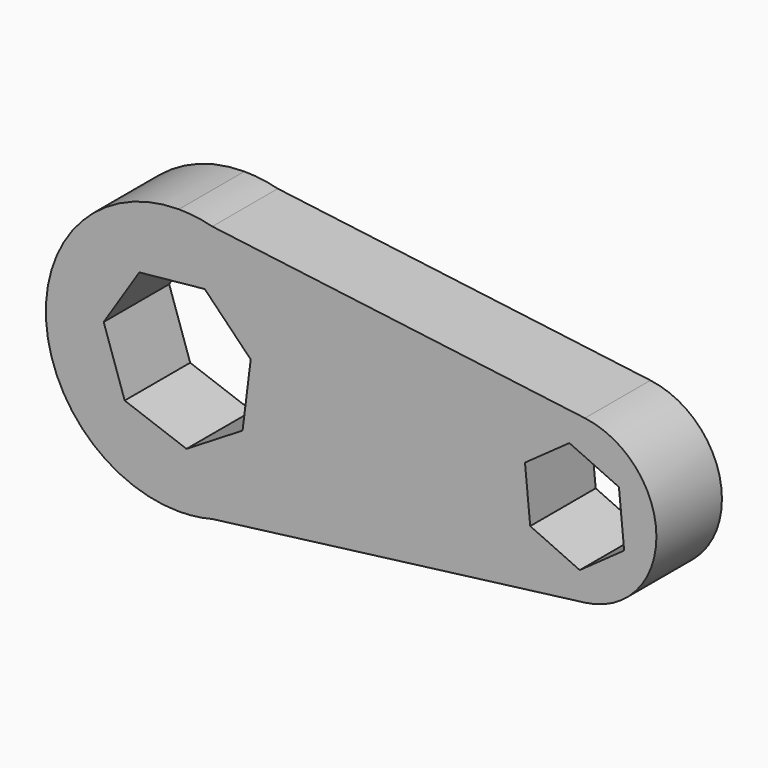
from build123d import *

# Parameters (mm, degrees)
F1_DEPTH = 50.8


# Not quite as in the source:
# - a feature names something its author has since deleted; it is built from what else it names


with BuildPart() as f1:
    # F0 (on Front) → F1 (new body)
    with BuildSketch(Plane.XZ):
        with BuildLine():
            Line((20.7350080501, 79.903453875), (0, 82.55))
            ThreePointArc((0, 82.55), (-82.55, 0), (0, -82.55))
            Line((0, -82.55), (20.7350080501, -79.903453875))
            ThreePointArc((20.7350080501, -79.903453875), (65.2923326836, -50.511521386), (82.55, 0))
            ThreePointArc((82.55, 0), (65.2923326836, 50.511521386), (20.7350080501, 79.903453875))
        make_face()
        Polygon((44.563520115, 15.0143387373), (39.5235830399, -25.4798759112), (4.7215818015, -46.7872243038), (-33.6358668361, -32.8628385102), (-46.6648216995, 5.8079349613), (-24.5542140343, 40.1052149467), (16.0462176134, 44.2024500799), align=None, mode=Mode.SUBTRACT)
        with BuildLine():
            ThreePointArc((20.7350080501, 79.903453875), (10.4516119, 81.8856905002), (0, 82.55))
            Line((0, 82.55), (20.7350080501, 79.903453875))
        make_face()
        with BuildLine():
            Line((20.7350080501, -79.903453875), (0, -82.55))
            ThreePointArc((0, -82.55), (10.4516119, -81.8856905002), (20.7350080501, -79.903453875))
        make_face()
        with BuildLine():
            Line((251.9559707698, 50.391194154), (20.7350080501, 79.903453875))
            ThreePointArc((20.7350080501, 79.903453875), (65.2923326836, 50.511521386), (82.55, 0))
            ThreePointArc((82.55, 0), (65.2923326836, -50.511521386), (20.7350080501, -79.903453875))
            Line((20.7350080501, -79.903453875), (251.9559707698, -50.391194154))
            ThreePointArc((251.9559707698, -50.391194154), (194.7242096006, 0), (251.9559707698, 50.391194154))
        make_face()
        with BuildLine():
            ThreePointArc((296.3242096006, 0), (283.6514535831, 33.5701246096), (251.9559707698, 50.391194154))
            ThreePointArc((251.9559707698, 50.391194154), (194.7242096006, 0), (251.9559707698, -50.391194154))
            ThreePointArc((251.9559707698, -50.391194154), (283.6514535831, -33.5701246096), (296.3242096006, 0))
        make_face()
        Polygon((273.0559987523, 19.6265456703), (276.2871913154, -14.0299559819), (248.7554021637, -33.6565016521), (217.9924204489, -19.6265456703), (214.7612278858, 14.0299559819), (242.2930170375, 33.6565016521), align=None, mode=Mode.SUBTRACT)
    extrude(amount=-F1_DEPTH)


solid = f1.part
